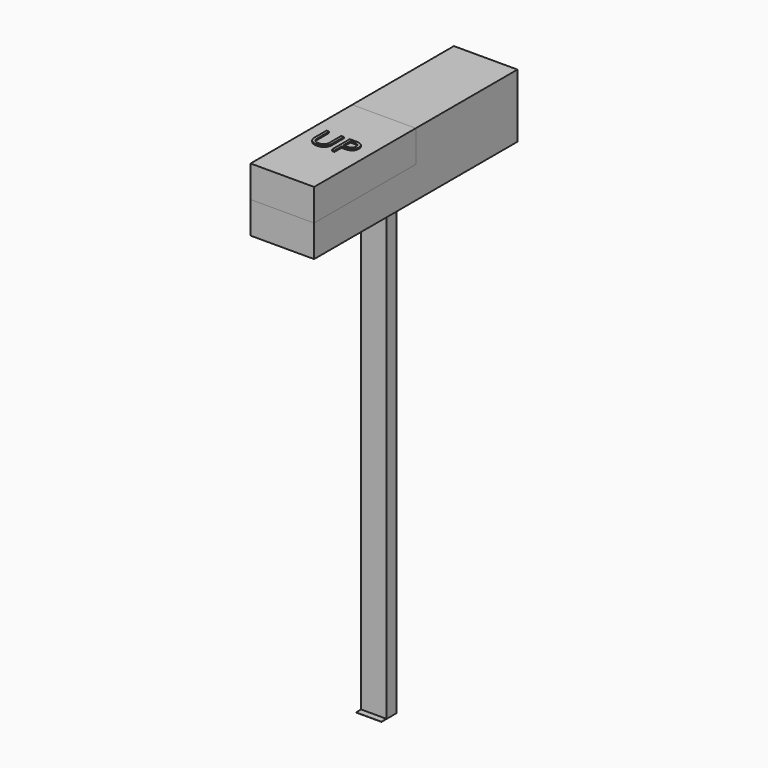
from build123d import *

# Parameters (mm, degrees)
F0_W          = 12.7
F0_H          = 12.7
F1_DEPTH      = 50.8
F2_W          = 25.4
F2_H          = 6.35
F3_DEPTH      = 25.4
F4_W          = 5.08
F4_H          = 2.54
F5_DEPTH      = 25.4
F6_W          = 25.4
F6_H          = 6.35
F7_DEPTH      = 12.7
F9_DEPTH      = 97.79
F10_W         = 5.08
F10_H         = 1.27
F11_DEPTH     = 0.0254
F12_TEXT_SIZE = 6.315859759
F13_DEPTH     = 0.254


# Not quite as in the source:
# - Text() gives the source's letters only with a copy of the font that has no kerning and outlines rounded to 1/6400 em; it was checked with that copy


with BuildPart() as f1:
    # F0 (on Front) → F1 (new body)
    with BuildSketch(Plane.XZ):
        Rectangle(F0_W, F0_H)
    extrude(amount=-F1_DEPTH)

    # F2 (on face) → F3 (cut)
    with BuildSketch(Plane.YZ.offset(6.35)):
        Polygon((-25.4, 0), (0, 0), (0, 6.35), (25.4, 6.35), (25.4, 12.7), (-25.4, 12.7), align=None)
        with Locations((12.7, 3.175)):
            Rectangle(F2_W, F2_H)
    extrude(amount=-F3_DEPTH, mode=Mode.SUBTRACT)

    # F4 (on face) → F5 (cut)
    with BuildSketch(Plane.XY):
        with Locations((0, 24.13)):
            Rectangle(F4_W, F4_H)
    extrude(amount=-F5_DEPTH, mode=Mode.SUBTRACT)


with BuildPart() as f7:
    # F6 (on face) → F7 (new body)
    with BuildSketch(Plane.YZ.offset(6.35)):
        with Locations((12.7, 3.175)):
            Rectangle(F6_W, F6_H)
    extrude(amount=-F7_DEPTH)

    # F8 (on face) → F9 (join)
    with BuildSketch(Plane(origin=(0, 0, 0), x_dir=(1, 0, 0), z_dir=(0, 0, -1))):
        Polygon((-2.54, -22.86), (-2.54, -25.4), (-1.27, -25.4), (1.27, -25.4), (2.54, -25.4), (2.54, -22.86), align=None)
    extrude(amount=F9_DEPTH)

    # F10 (on face) → F11 (join)
    with BuildSketch(Plane(origin=(0, 0, -97.79), x_dir=(1, 0, 0), z_dir=(0, 0, -1))):
        with Locations((0, -22.225)):
            Rectangle(F10_W, F10_H)
    extrude(amount=-F11_DEPTH)

    # F12 (on face) → F13 (join)
    with BuildSketch(Plane.XY.offset(6.35)):
        with Locations((-4.3016126001, 11.2046767026)):
            Text('UP', F12_TEXT_SIZE, font='Open Sans', text_align=(TextAlign.LEFT, TextAlign.BOTTOM))
    extrude(amount=F13_DEPTH)


solid = Compound([f1.part, f7.part])
